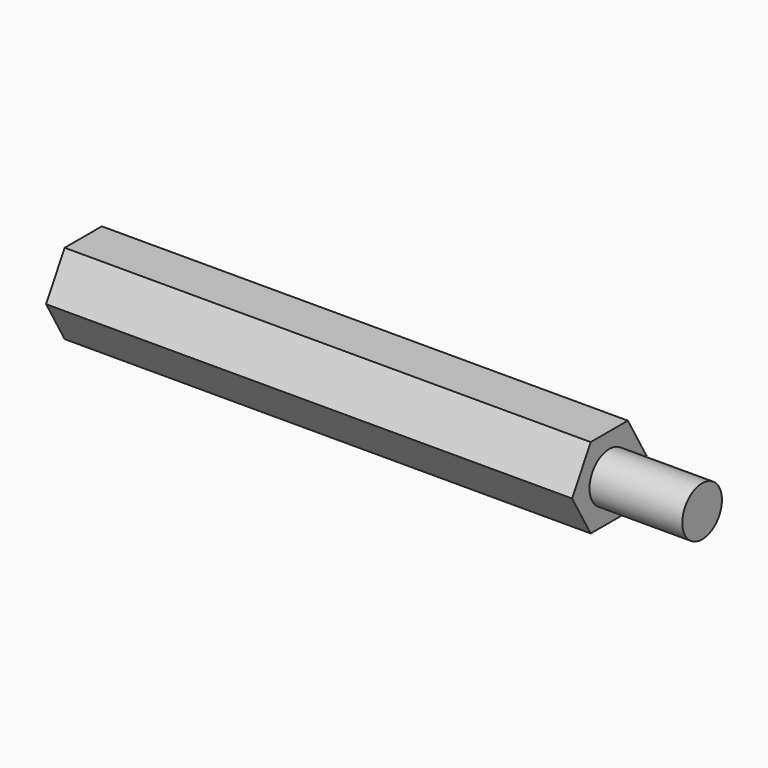
from build123d import *

# Parameters (mm, degrees)
F0_R     = 4
F0_R_2   = 3
F1_DEPTH = 85
F2_DEPTH = 25
F3_START = 85
F3_DEPTH = 15


# Not quite as in the source:
# - a feature names something its author has since deleted; it is built from what else it names


with BuildPart() as f1:
    # F0 (on Right) → F1 (new body)
    with BuildSketch(Plane.YZ):
        Polygon((-3.7528207105, 6.4999746191), (-7.5055534993, -5.07616e-05), (-3.7527327888, -6.5000253806), (3.7528207105, -6.4999746191), (7.5055534993, 5.07616e-05), (3.7527327888, 6.5000253806), align=None)
        Circle(F0_R, mode=Mode.SUBTRACT)
        Circle(F0_R)
        Circle(F0_R_2, mode=Mode.SUBTRACT)
        Circle(F0_R_2)
    extrude(amount=F1_DEPTH)

    # F0 (on Right) → F2 (cut)
    with BuildSketch(Plane.YZ):
        Circle(F0_R_2)
    extrude(amount=F2_DEPTH, mode=Mode.SUBTRACT)

    # F0 (on Right) → F3 (join)
    with BuildSketch(Plane.YZ.offset(F3_START)):
        Circle(F0_R)
        Circle(F0_R_2, mode=Mode.SUBTRACT)
        Circle(F0_R_2)
    extrude(amount=F3_DEPTH)


solid = f1.part
